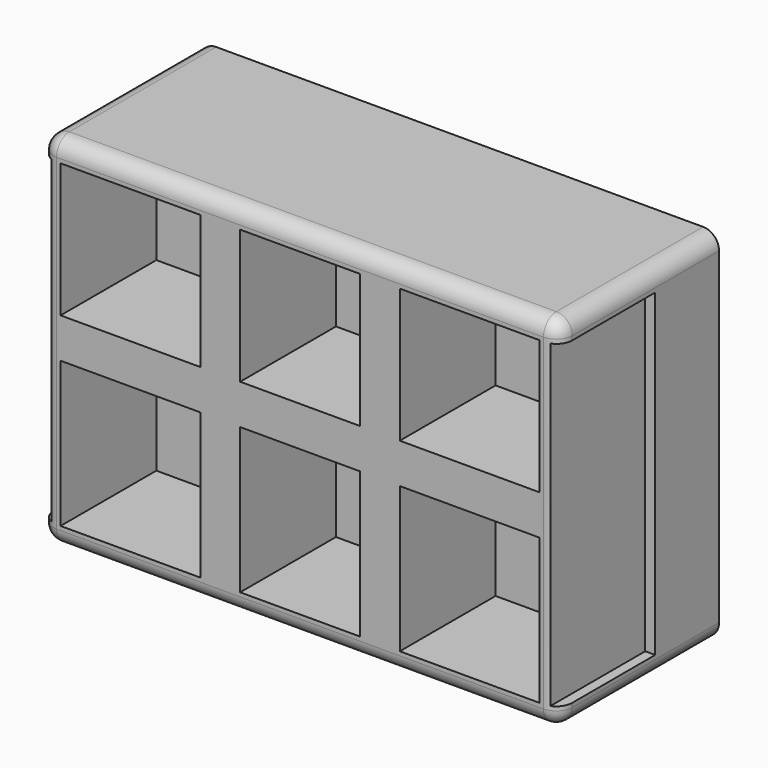
from build123d import *

# Parameters (mm, degrees)
F0_W     = 3.175
F0_H     = 6.35
F0_W_2   = 6.35
F0_W_3   = 44.45
F0_W_4   = 15.0601655953
F0_W_5   = 5.811475683
F0_W_6   = 6.888524317
F0_W_7   = 10.3398344047
F0_H_2   = 42.6130002154
F0_H_3   = 46.2869997846
F1_DEPTH = 50.8
F0_H_4   = 52.6369997846
F0_H_5   = 48.9630002154
F2_DEPTH = 12.7
F3_F1_R  = 5.08
F3_F2_R  = 5.08
F3_F3_R  = 5.08
F3_F4_R  = 5.08


with BuildPart() as f1:
    # F0 (on Front) → F1 (new body)
    with BuildSketch(Plane.XZ):
        Polygon((0, -58.9869997846), (0, -52.6369997846), (-5.811475683, -52.6369997846), (-20.8716412783, -52.6369997846), (-27.2216412783, -52.6369997846), (-33.5716412783, -52.6369997846), (-78.0216412783, -52.6369997846), (-78.0216412783, -58.9869997846), align=None)
        with Locations((-79.6091412783, 52.1380002154)):
            Rectangle(F0_W, F0_H)
        with Locations((-82.7841412783, 52.1380002154)):
            Rectangle(F0_W, F0_H)
        Polygon((-5.811475683, 48.9630002154), (0, 48.9630002154), (0, 55.3130002154), (-78.0216412783, 55.3130002154), (-78.0216412783, 48.9630002154), (-33.5716412783, 48.9630002154), (-27.2216412783, 48.9630002154), (-20.8716412783, 48.9630002154), align=None)
        Polygon((0, 55.3130002154), (0, 48.9630002154), (6.888524317, 48.9630002154), (17.2283587217, 48.9630002154), (23.5783587217, 48.9630002154), (29.9283587217, 48.9630002154), (74.3783587217, 48.9630002154), (74.3783587217, 55.3130002154), align=None)
        Polygon((80.7283587217, 55.3130002154), (77.5533587217, 55.3130002154), (77.5533587217, 48.9315246976), (80.7283587217, 48.9000491798), align=None)
        Polygon((77.5533587217, 55.3130002154), (74.3783587217, 55.3130002154), (74.3783587217, 48.9630002154), (77.5533587217, 48.9315246976), align=None)
        Polygon((6.888524317, -52.6369997846), (0, -52.6369997846), (0, -58.9869997846), (80.7283587217, -58.9869997846), (80.7283587217, -52.6369997846), (77.5533587217, -52.6369997846), (74.3783587217, -52.6369997846), (29.9283587217, -52.6369997846), (23.5783587217, -52.6369997846), (17.2283587217, -52.6369997846), align=None)
        with Locations((-82.7841412783, -55.8119997846)):
            Rectangle(F0_W, F0_H)
        with Locations((-79.6091412783, -55.8119997846)):
            Rectangle(F0_W, F0_H)
        with Locations((-30.3966412783, 3.175)):
            Rectangle(F0_W_2, F0_H)
        with Locations((-24.0466412783, 3.175)):
            Rectangle(F0_W_2, F0_H)
        with Locations((-30.3966412783, -3.175)):
            Rectangle(F0_W_2, F0_H)
        with Locations((-24.0466412783, -3.175)):
            Rectangle(F0_W_2, F0_H)
        with Locations((20.4033587217, -3.175)):
            Rectangle(F0_W_2, F0_H)
        with Locations((20.4033587217, 3.175)):
            Rectangle(F0_W_2, F0_H)
        with Locations((26.7533587217, 3.175)):
            Rectangle(F0_W_2, F0_H)
        with Locations((26.7533587217, -3.175)):
            Rectangle(F0_W_2, F0_H)
        with Locations((-55.7966412783, 3.175)):
            Rectangle(F0_W_3, F0_H)
        with Locations((-55.7966412783, -3.175)):
            Rectangle(F0_W_3, F0_H)
        with Locations((-13.3415584806, 3.175)):
            Rectangle(F0_W_4, F0_H)
        with Locations((-13.3415584806, -3.175)):
            Rectangle(F0_W_4, F0_H)
        with Locations((-2.9057378415, 3.175)):
            Rectangle(F0_W_5, F0_H)
        with Locations((-2.9057378415, -3.175)):
            Rectangle(F0_W_5, F0_H)
        with Locations((3.4442621585, -3.175)):
            Rectangle(F0_W_6, F0_H)
        with Locations((3.4442621585, 3.175)):
            Rectangle(F0_W_6, F0_H)
        with Locations((12.0584415194, -3.175)):
            Rectangle(F0_W_7, F0_H)
        with Locations((12.0584415194, 3.175)):
            Rectangle(F0_W_7, F0_H)
        with Locations((52.1533587217, 3.175)):
            Rectangle(F0_W_3, F0_H)
        with Locations((52.1533587217, -3.175)):
            Rectangle(F0_W_3, F0_H)
        with Locations((-30.3966412783, 27.6565001077)):
            Rectangle(F0_W_2, F0_H_2)
        with Locations((-24.0466412783, 27.6565001077)):
            Rectangle(F0_W_2, F0_H_2)
        with Locations((-30.3966412783, -29.4934998923)):
            Rectangle(F0_W_2, F0_H_3)
        with Locations((-24.0466412783, -29.4934998923)):
            Rectangle(F0_W_2, F0_H_3)
        with Locations((20.4033587217, 27.6565001077)):
            Rectangle(F0_W_2, F0_H_2)
        with Locations((26.7533587217, 27.6565001077)):
            Rectangle(F0_W_2, F0_H_2)
        with Locations((20.4033587217, -29.4934998923)):
            Rectangle(F0_W_2, F0_H_3)
        with Locations((26.7533587217, -29.4934998923)):
            Rectangle(F0_W_2, F0_H_3)
        Polygon((77.5533587217, 48.9315246976), (74.3783587217, 48.9630002154), (74.3783587217, 6.35), (74.3783587217, 0), (77.5533587217, 0), align=None)
        Polygon((77.5533587217, 0), (74.3783587217, 0), (74.3783587217, -6.35), (74.3783587217, -52.6369997846), (77.5533587217, -52.6369997846), align=None)
        Polygon((-78.0216412783, 6.35), (-78.0216412783, 48.9630002154), (-81.1966412783, 48.9630002154), (-81.1966412783, 0), (-78.0216412783, 0), align=None)
        Polygon((-81.1966412783, -52.6369997846), (-78.0216412783, -52.6369997846), (-78.0216412783, -6.35), (-78.0216412783, 0), (-81.1966412783, 0), align=None)
    extrude(amount=F1_DEPTH)

    # F0 (on Front) → F2 (join, symmetric)
    with BuildSketch(Plane.XZ):
        with Locations((-2.9057378415, 3.175)):
            Rectangle(F0_W_5, F0_H)
        with Locations((3.4442621585, -3.175)):
            Rectangle(F0_W_6, F0_H)
        with Locations((-2.9057378415, -3.175)):
            Rectangle(F0_W_5, F0_H)
        with Locations((3.4442621585, 3.175)):
            Rectangle(F0_W_6, F0_H)
        with Locations((-2.9057378415, 27.6565001077)):
            Rectangle(F0_W_5, F0_H_2)
        with Locations((3.4442621585, 27.6565001077)):
            Rectangle(F0_W_6, F0_H_2)
        with Locations((3.4442621585, -29.4934998923)):
            Rectangle(F0_W_6, F0_H_3)
        with Locations((-2.9057378415, -29.4934998923)):
            Rectangle(F0_W_5, F0_H_3)
        with Locations((-13.3415584806, -3.175)):
            Rectangle(F0_W_4, F0_H)
        with Locations((-13.3415584806, 3.175)):
            Rectangle(F0_W_4, F0_H)
        with Locations((12.0584415194, 3.175)):
            Rectangle(F0_W_7, F0_H)
        with Locations((12.0584415194, -3.175)):
            Rectangle(F0_W_7, F0_H)
        Polygon((0, 55.3130002154), (0, 48.9630002154), (6.888524317, 48.9630002154), (17.2283587217, 48.9630002154), (23.5783587217, 48.9630002154), (29.9283587217, 48.9630002154), (74.3783587217, 48.9630002154), (74.3783587217, 55.3130002154), align=None)
        Polygon((-5.811475683, 48.9630002154), (0, 48.9630002154), (0, 55.3130002154), (-78.0216412783, 55.3130002154), (-78.0216412783, 48.9630002154), (-33.5716412783, 48.9630002154), (-27.2216412783, 48.9630002154), (-20.8716412783, 48.9630002154), align=None)
        with Locations((12.0584415194, 27.6565001077)):
            Rectangle(F0_W_7, F0_H_2)
        with Locations((-13.3415584806, 27.6565001077)):
            Rectangle(F0_W_4, F0_H_2)
        Polygon((0, -58.9869997846), (0, -52.6369997846), (-5.811475683, -52.6369997846), (-20.8716412783, -52.6369997846), (-27.2216412783, -52.6369997846), (-33.5716412783, -52.6369997846), (-78.0216412783, -52.6369997846), (-78.0216412783, -58.9869997846), align=None)
        Polygon((6.888524317, -52.6369997846), (0, -52.6369997846), (0, -58.9869997846), (80.7283587217, -58.9869997846), (80.7283587217, -52.6369997846), (77.5533587217, -52.6369997846), (74.3783587217, -52.6369997846), (29.9283587217, -52.6369997846), (23.5783587217, -52.6369997846), (17.2283587217, -52.6369997846), align=None)
        with Locations((12.0584415194, -29.4934998923)):
            Rectangle(F0_W_7, F0_H_3)
        with Locations((-13.3415584806, -29.4934998923)):
            Rectangle(F0_W_4, F0_H_3)
        with Locations((-79.6091412783, 52.1380002154)):
            Rectangle(F0_W, F0_H)
        Polygon((77.5533587217, 55.3130002154), (74.3783587217, 55.3130002154), (74.3783587217, 48.9630002154), (77.5533587217, 48.9315246976), align=None)
        with Locations((-79.6091412783, -55.8119997846)):
            Rectangle(F0_W, F0_H)
        with Locations((-55.7966412783, 27.6565001077)):
            Rectangle(F0_W_3, F0_H_2)
        with Locations((-82.7841412783, 52.1380002154)):
            Rectangle(F0_W, F0_H)
        with Locations((52.1533587217, 27.6565001077)):
            Rectangle(F0_W_3, F0_H_2)
        Polygon((80.7283587217, 55.3130002154), (77.5533587217, 55.3130002154), (77.5533587217, 48.9315246976), (80.7283587217, 48.9000491798), align=None)
        with Locations((79.1408587217, -26.3184998923)):
            Rectangle(F0_W, F0_H_4)
        with Locations((-55.7966412783, -29.4934998923)):
            Rectangle(F0_W_3, F0_H_3)
        with Locations((-82.7841412783, -55.8119997846)):
            Rectangle(F0_W, F0_H)
        with Locations((52.1533587217, -29.4934998923)):
            Rectangle(F0_W_3, F0_H_3)
        with Locations((-82.7841412783, 24.4815001077)):
            Rectangle(F0_W, F0_H_5)
        Polygon((80.7283587217, 48.9000491798), (77.5533587217, 48.9315246976), (77.5533587217, 0), (80.7283587217, 0), align=None)
        with Locations((-82.7841412783, -26.3184998923)):
            Rectangle(F0_W, F0_H_4)
    extrude(amount=F2_DEPTH, both=True)

    # F3: fillet of radius 5.08 on 10 edges, made by hand

    # F3_f1
    f3_f1_edges = [f1.edges().sort_by_distance(p)[0] for p in [
        (80.7283587217, -19.05, 55.3130002154),
    ]]
    fillet(f3_f1_edges, radius=F3_F1_R)

    # F3_f2
    f3_f2_edges = [f1.edges().sort_by_distance(p)[0] for p in [
        (-84.3716412783, -19.05, 55.3130002154),
    ]]
    fillet(f3_f2_edges, radius=F3_F2_R)

    # F3_f3
    f3_f3_edges = [f1.edges().sort_by_distance(p)[0] for p in [
        (-1.8216412783, -50.8, 55.3130002154),
    ]]
    fillet(f3_f3_edges, radius=F3_F3_R)

    # F3_f4
    f3_f4_edges = [f1.edges().sort_by_distance(p)[0] for p in [
        (-1.8216412783, -50.8, -58.9869997846),
    ]]
    fillet(f3_f4_edges, radius=F3_F4_R)


solid = f1.part
